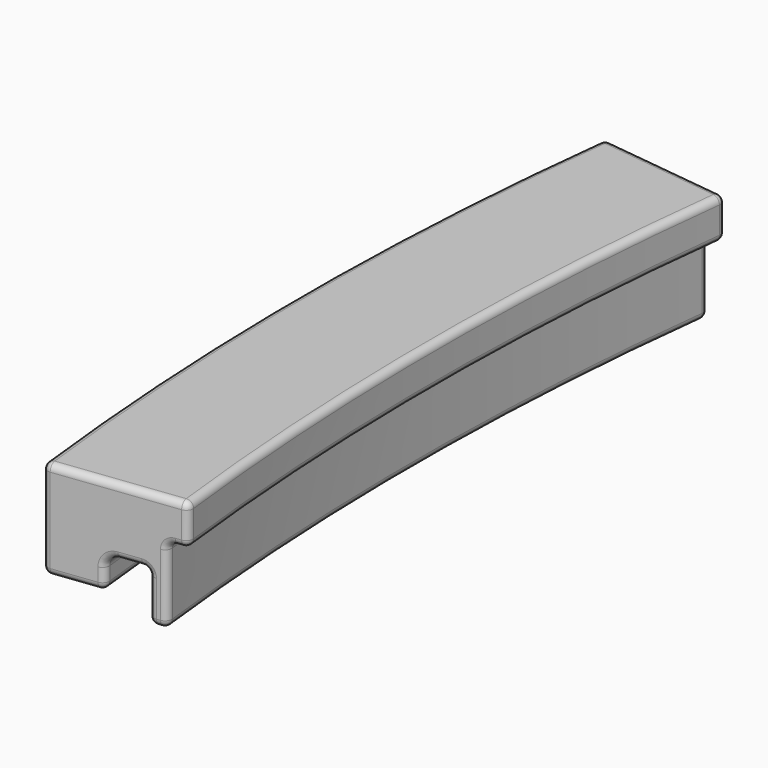
from build123d import *

# Parameters (mm, degrees)
F4_R = 2.54
F5_R = 1.4986


# Not quite as in the source:
# - a feature names something its author has since deleted; it is built from what else it names


with BuildPart() as f2:
    # F2: sweep along a path in F1
    with BuildLine(Plane.XY) as f2_path:
        ThreePointArc((-3.4654962667, 76.2), (-6.9058923043, 38.1690157564), (-8.0540750503, 0))
    # F0 (on Front) → F2 (sweep)
    with BuildSketch(Plane.XZ):
        Polygon((-20.7540750503, 7.305548638), (-20.7540750503, -14.4514460401), (-16.9440750503, -14.4514460401), (-11.8640750503, -14.4514460401), (-8.0540750503, -14.4514460401), (-8.0540750503, -7.4444001753), (0.8359249497, -7.4444001753), (0.8359249497, -18.3827867696), (4.6459249497, -18.3827867696), (4.6459249497, -1.584451362), (8.9475380868, -1.584451362), (8.9475380868, 7.305548638), align=None)
    sweep(path=f2_path.line)

    # F3: F2 across plane


with BuildPart() as f2_1:
    add(f2.part)
    add(f2.part.mirror(Plane.XZ))

    # F4
    f4_edges = [f2_1.edges().sort_by_distance(p)[0] for p in [
        (-8.054075, 0, -7.4444),
    ]]
    fillet(f4_edges, radius=F4_R)

    # F5
    f5_edges = [f2_1.edges().sort_by_distance(p)[0] for p in [
        (0.835925, 0, -7.4444),
        (4.645925, 0, -18.382787),
        (0.835925, 0, -18.382787),
        (4.645925, 0, -1.584451),
        (7.251498, -74.9046, -18.382787),
        (7.251498, 74.9046, -18.382787),
        (5.360264, 75.1332, -12.913593),
        (5.360264, -75.1332, -12.913593),
        (9.142732, -74.676, -9.983619),
        (8.947538, 0, -1.584451),
        (9.142732, 74.676, -9.983619),
        (13.413261, -74.159806, 2.860549),
        (8.947538, 0, 7.305549),
        (-1.330232, -75.941903, 7.305549),
        (-16.073725, -77.724, -3.572949),
        (-20.754075, 0, 7.305549),
        (-9.76961, -76.962, -14.451446),
        (-8.054075, 0, -14.451446),
        (-20.754075, 0, -14.451446),
        (-9.76961, 76.962, -14.451446),
        (-16.073725, 77.724, -3.572949),
        (-1.330232, 75.941903, 7.305549),
        (13.413261, 74.159806, 2.860549),
        (-3.465496, 76.2, -12.217923),
        (-2.726923, 76.110726, -8.188349),
        (2.208207, 75.5142, -7.4444),
        (11.277997, 74.417903, -1.584451),
        (-3.465496, -76.2, -12.217923),
        (-2.726923, -76.110726, -8.188349),
        (2.208207, -75.5142, -7.4444),
        (11.277997, -74.417903, -1.584451),
    ]]
    fillet(f5_edges, radius=F5_R)


solid = f2_1.part
